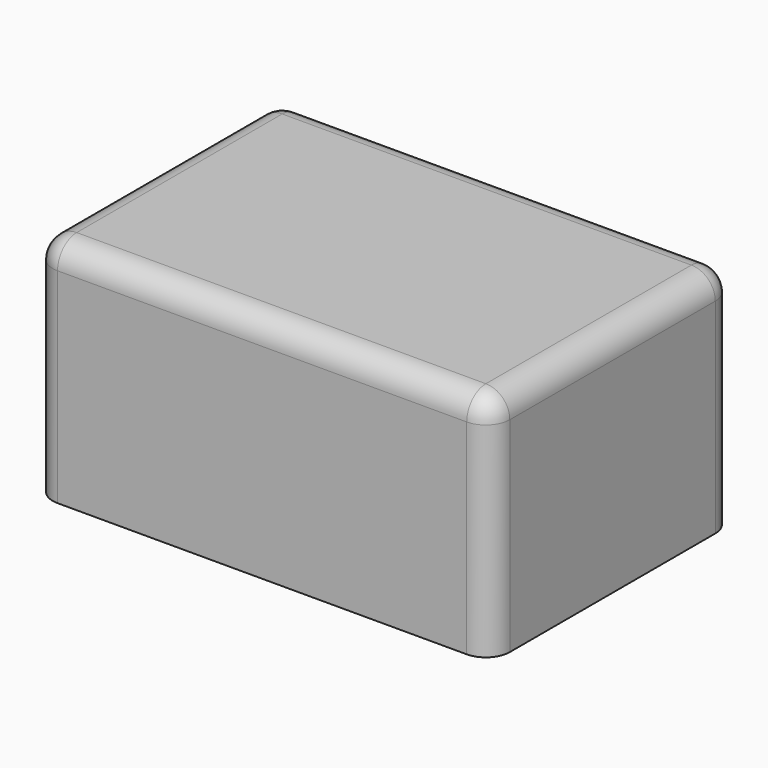
from build123d import *

# Parameters (mm, degrees)
F0_W         = 60
F0_H         = 40
F0_W_2       = 56
F0_H_2       = 36
F1_DEPTH     = 30
F2_DEPTH     = 28
F3_R         = 3.1384776311
F6_W         = 56
F6_H         = 1.5
F7_DEPTH     = 1
F5_W         = 56
F5_H         = 1.5
F8_DEPTH     = 1
F9_W         = 2
F9_H         = 36
F10_DEPTH    = 3.1
F6_W_2       = 2
F11_DEPTH    = 1
F5_W_2       = 2
F12_DEPTH    = 1
F4_TEXT_SIZE = 10.7436629176
F13_DEPTH    = 1


# Not quite as in the source:
# - Text() gives the source's letters only with a copy of the font that has no kerning and outlines rounded to 1/6400 em; it was checked with that copy


with BuildPart() as f1:
    # F0 (on Top) → F1 (new body)
    with BuildSketch(Plane.XY):
        Rectangle(F0_W, F0_H)
        Rectangle(F0_W_2, F0_H_2, mode=Mode.SUBTRACT)
        Rectangle(F0_W_2, F0_H_2)
    extrude(amount=F1_DEPTH)

    # F0 (on Top) → F2 (cut)
    with BuildSketch(Plane.XY):
        Rectangle(F0_W_2, F0_H_2)
    extrude(amount=F2_DEPTH, mode=Mode.SUBTRACT)

    # F3
    f3_edges = [f1.edges().sort_by_distance(p)[0] for p in [
        (30, -20, 15),
        (30, 0, 30),
        (30, 20, 15),
        (0, 20, 30),
        (-30, 20, 15),
        (-30, 0, 30),
        (-30, -20, 15),
        (0, -20, 30),
    ]]
    fillet(f3_edges, radius=F3_R)

    # F6 (on face) → F7 (cut)
    with BuildSketch(Plane(origin=(0, -18, 0), x_dir=(-1, 0, 0), z_dir=(0, 1, 0))):
        with Locations((0, 2.25)):
            Rectangle(F6_W, F6_H)
    extrude(amount=-F7_DEPTH, mode=Mode.SUBTRACT)

    # F5 (on face) → F8 (cut)
    with BuildSketch(Plane.XZ.offset(-18)):
        with Locations((0, 2.25)):
            Rectangle(F5_W, F5_H)
    extrude(amount=-F8_DEPTH, mode=Mode.SUBTRACT)

    # F9 (on face) → F10 (cut)
    with BuildSketch(Plane(origin=(0, 0, 0), x_dir=(1, 0, 0), z_dir=(0, 0, -1))):
        with Locations((-29, 0)):
            Rectangle(F9_W, F9_H)
    extrude(amount=-F10_DEPTH, mode=Mode.SUBTRACT)

    # F6 (on face) → F11 (cut)
    with BuildSketch(Plane(origin=(0, -18, 0), x_dir=(-1, 0, 0), z_dir=(0, 1, 0))):
        with Locations((29, 2.25)):
            Rectangle(F6_W_2, F6_H)
    extrude(amount=-F11_DEPTH, mode=Mode.SUBTRACT)

    # F5 (on face) → F12 (cut)
    with BuildSketch(Plane.XZ.offset(-18)):
        with Locations((-29, 2.25)):
            Rectangle(F5_W_2, F5_H)
    extrude(amount=-F12_DEPTH, mode=Mode.SUBTRACT)

    # F4 (on face) → F13 (join)
    with BuildSketch(Plane(origin=(0, 20, 0), x_dir=(-1, 0, 0), z_dir=(0, 1, 0))):
        with Locations((-24.9159545099, 14.1260850683)):
            Text('Edderboks', F4_TEXT_SIZE, font='Open Sans', font_style=FontStyle.ITALIC, text_align=(TextAlign.LEFT, TextAlign.BOTTOM))
    extrude(amount=F13_DEPTH)


solid = f1.part
